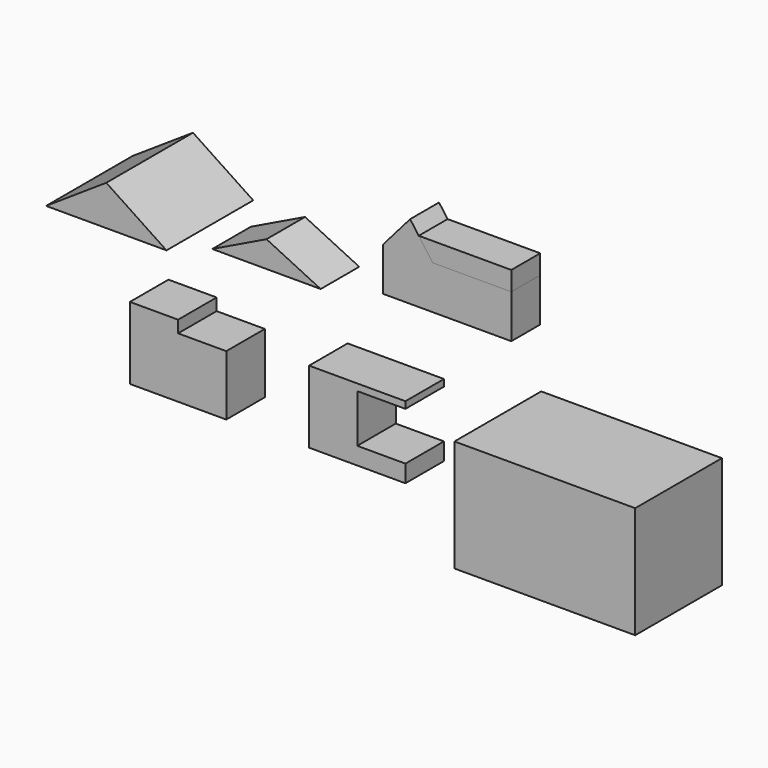
from build123d import *

# Parameters (mm, degrees)
F1_DEPTH  = 127
F4_DEPTH  = 76.2
F6_DEPTH  = 25.4
F8_DEPTH  = 101.6
F9_W      = 165.6684279442
F9_H      = 91.7260497808
F11_DEPTH = 76.2
F13_DEPTH = 101.6
F14_W     = 101.6
F14_H     = 101.6
F15_DEPTH = 101.6
F16_W     = 101.6
F16_H     = 101.6
F17_DEPTH = 127
F18_W     = 381.1446428299
F18_H     = 235.9467148781
F20_DEPTH = 127
F21_W     = 381.1446428299
F21_H     = 235.9467148781
F19_W     = 381.1446428299
F19_H     = 235.9467148781
F23_DEPTH = 101.6


with BuildPart() as f1:
    # F0 (on Front) → F1 (new body)
    with BuildSketch(Plane.XZ):
        Polygon((195.0628506741, 48.968303573), (68.0628506741, -35.273966102), (322.0628506741, -35.273966102), align=None)
    extrude(amount=F1_DEPTH)

    # F2 (on face) → F4 (join)
    with BuildSketch(Plane.XZ.offset(127)):
        Polygon((68.0628506741, -35.273966102), (322.0628506741, -35.273966102), (195.0628506741, 48.968303573), align=None)
    extrude(amount=F4_DEPTH)

    # F5 (on face) → F6 (join)
    with BuildSketch(Plane.XZ.offset(203.2)):
        Polygon((195.0628506741, 48.968303573), (68.0628506741, -35.273966102), (322.0628506741, -35.273966102), align=None)
    extrude(amount=F6_DEPTH)


with BuildPart() as f8:
    # F7 (on Front) → F8 (new body)
    with BuildSketch(Plane.XZ):
        Polygon((545.6249140978, -85.9377876582), (431.3249140978, -30.5797710753), (317.0249140978, -85.9377876582), align=None)
    extrude(amount=F8_DEPTH)


with BuildPart() as f11:
    # F9 (on Front) → F11 (new body)
    with BuildSketch(Plane.XZ):
        with Locations((844.5067703724, -23.1638774276)):
            Rectangle(F9_W, F9_H)
        Polygon((713.9375209808, 88.2177501917), (656.8427681923, 22.6991474628), (656.8427681923, -69.026902318), (761.6725564003, -69.026902318), (761.6725564003, 22.6991474628), (732.0935192904, 63.2977804056), align=None)
    extrude(amount=F11_DEPTH)


with BuildPart() as f11b:
    # F10 (on face) → F11, piece 2 (new body)
    with BuildSketch(Plane.XZ):
        Polygon((927.3409843445, 22.6991474628), (927.3409843445, 63.2977804056), (732.0935192904, 63.2977804056), (761.6725564003, 22.6991474628), align=None)
    extrude(amount=F11_DEPTH)


with BuildPart() as f13:
    # F12 (on Front) → F13 (new body)
    with BuildSketch(Plane.XZ):
        Polygon((244.8786242905, -240.6501034379), (143.2786242905, -240.6501034379), (143.2786242905, -393.0501034379), (346.4786242905, -393.0501034379), (346.4786242905, -266.0501034379), (244.8786242905, -266.0501034379), align=None)
    extrude(amount=F13_DEPTH)


with BuildPart() as f15:
    # F14 (on Front) → F15 (new body)
    with BuildSketch(Plane.XZ):
        Polygon((724.3456629276, -236.1136930588), (521.1456629276, -236.1136930588), (521.1456629276, -388.5136930588), (724.3456629276, -388.5136930588), (724.3456629276, -360.9611363416), (622.7456629276, -360.9611363416), (622.7456629276, -259.3611363416), (724.3456629276, -259.3611363416), align=None)
        with Locations((673.5456629276, -310.1611363416)):
            Rectangle(F14_W, F14_H)
    extrude(amount=F15_DEPTH)

    # F16 (on face) → F17 (cut)
    with BuildSketch(Plane.XZ.offset(101.6)):
        with Locations((673.5456629276, -301.1498109818)):
            Rectangle(F16_W, F16_H)
    extrude(amount=-F17_DEPTH, mode=Mode.SUBTRACT)


with BuildPart() as f20:
    # F18 (on Front) → F20 (new body)
    with BuildSketch(Plane.XZ):
        with Locations((1119.9880242348, -310.4507923126)):
            Rectangle(F18_W, F18_H)
    extrude(amount=F20_DEPTH)

    # F21 (on face) + F19 (on face) → F23 (join)
    with BuildSketch(Plane.XZ.offset(127)):
        with Locations((1119.9880242348, -310.4507923126)):
            Rectangle(F21_W, F21_H)
    with BuildSketch(Plane.XZ):
        with Locations((1119.9880242348, -310.4507923126)):
            Rectangle(F19_W, F19_H)
    extrude(amount=F23_DEPTH)


solid = Compound([f1.part, f8.part, f11.part, f11b.part, f13.part, f15.part, f20.part])
